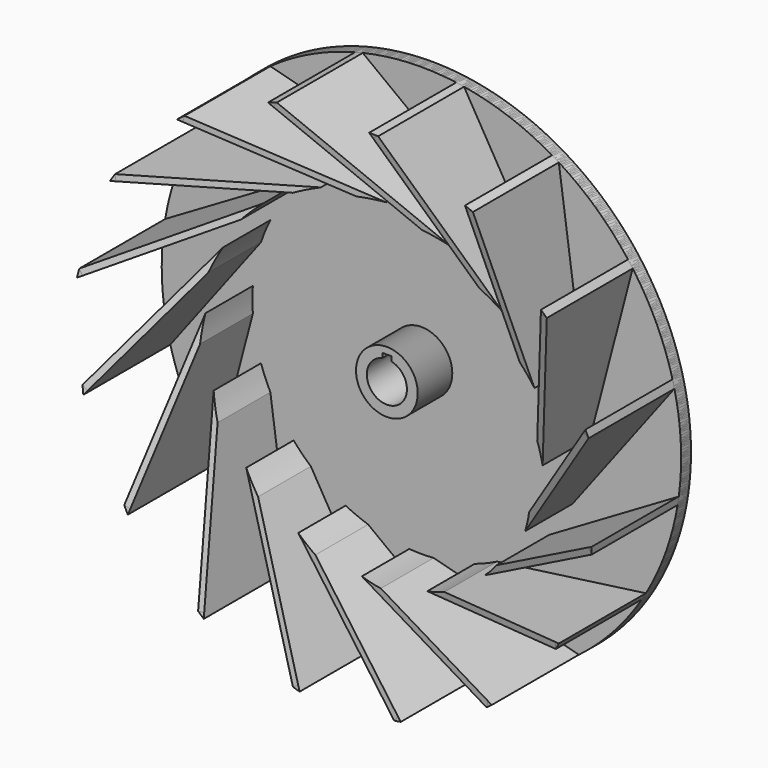
from build123d import *

# Parameters (mm, degrees)
F0_R      = 267.335
F0_R_2    = 20.6375
F1_DEPTH  = 12.7
F3_DEPTH  = 241.3
F2_R      = 31.75
F2_R_2    = 20.6375
F4_DEPTH  = 44.45
F7_DEPTH  = 6.35
F8_COUNT  = 16
F10_DEPTH = 57.15


# Not quite as in the source:
# - a feature names something its author has since deleted; it is built from what else it names


with BuildPart() as f1:
    # F0 (on Front) → F1 (new body)
    with BuildSketch(Plane.XZ):
        Circle(F0_R)
        Circle(F0_R_2, mode=Mode.SUBTRACT)
    extrude(amount=F1_DEPTH)

    # F2 (on face) → F3 (join)
    with BuildSketch(Plane.XZ.offset(12.7)):
        with BuildLine():
            Line((-162.0244501567, 212.6407293451), (-12.5453111688, 173.5371293634))
            ThreePointArc((-12.5453111688, 173.5371293634), (0, 173.99), (12.5453111688, 173.5371293634))
            Line((12.5453111688, 173.5371293634), (-155.4588853582, 217.4868667028))
            ThreePointArc((-155.4588853582, 217.4868667028), (-158.7601598142, 215.0888511308), (-162.0244501567, 212.6407293451))
        make_face()
    extrude(amount=F3_DEPTH)

    # F2 (on face) → F4 (join)
    with BuildSketch(Plane.XZ.offset(12.7)):
        Circle(F2_R)
        Circle(F2_R_2, mode=Mode.SUBTRACT)
    extrude(amount=F4_DEPTH)

    # F5 (on face) → F7 (cut, through all)
    with BuildSketch(Plane(origin=(43.2929607784, 0, 165.4935735946), x_dir=(0.9674446735, 0, -0.2530826025), z_dir=(0.2530826025, 0, 0.9674446735))):
        Polygon((-205.4400128284, -123.2503851183), (-205.4400128284, -254), (-31.7823338652, -254), (-31.7823338652, -73.66), align=None)
        Polygon((-210.5653604666, -124.714), (-210.5653604666, -254), (-205.4400128284, -254), (-205.4400128284, -123.2503851183), align=None)
    extrude(amount=-F7_DEPTH, mode=Mode.SUBTRACT)


with BuildPart() as f8_1:
    # F8: instance of F1
    add(f1.part.rotate(Axis((0, -75.4788592458, 0), (0, -1, 0)), 1 * 360 / F8_COUNT))


with BuildPart() as f8_2:
    # F8: instance of F1
    add(f1.part.rotate(Axis((0, -75.4788592458, 0), (0, -1, 0)), 2 * 360 / F8_COUNT))


with BuildPart() as f8_3:
    # F8: instance of F1
    add(f1.part.rotate(Axis((0, -75.4788592458, 0), (0, -1, 0)), 3 * 360 / F8_COUNT))


with BuildPart() as f8_4:
    # F8: instance of F1
    add(f1.part.rotate(Axis((0, -75.4788592458, 0), (0, -1, 0)), 4 * 360 / F8_COUNT))


with BuildPart() as f8_5:
    # F8: instance of F1
    add(f1.part.rotate(Axis((0, -75.4788592458, 0), (0, -1, 0)), 5 * 360 / F8_COUNT))


with BuildPart() as f8_6:
    # F8: instance of F1
    add(f1.part.rotate(Axis((0, -75.4788592458, 0), (0, -1, 0)), 6 * 360 / F8_COUNT))


with BuildPart() as f8_7:
    # F8: instance of F1
    add(f1.part.rotate(Axis((0, -75.4788592458, 0), (0, -1, 0)), 7 * 360 / F8_COUNT))


with BuildPart() as f8_8:
    # F8: instance of F1
    add(f1.part.rotate(Axis((0, -75.4788592458, 0), (0, -1, 0)), 8 * 360 / F8_COUNT))


with BuildPart() as f8_9:
    # F8: instance of F1
    add(f1.part.rotate(Axis((0, -75.4788592458, 0), (0, -1, 0)), 9 * 360 / F8_COUNT))


with BuildPart() as f8_10:
    # F8: instance of F1
    add(f1.part.rotate(Axis((0, -75.4788592458, 0), (0, -1, 0)), 10 * 360 / F8_COUNT))


with BuildPart() as f8_11:
    # F8: instance of F1
    add(f1.part.rotate(Axis((0, -75.4788592458, 0), (0, -1, 0)), 11 * 360 / F8_COUNT))


with BuildPart() as f8_12:
    # F8: instance of F1
    add(f1.part.rotate(Axis((0, -75.4788592458, 0), (0, -1, 0)), 12 * 360 / F8_COUNT))


with BuildPart() as f8_13:
    # F8: instance of F1
    add(f1.part.rotate(Axis((0, -75.4788592458, 0), (0, -1, 0)), 13 * 360 / F8_COUNT))


with BuildPart() as f8_14:
    # F8: instance of F1
    add(f1.part.rotate(Axis((0, -75.4788592458, 0), (0, -1, 0)), 14 * 360 / F8_COUNT))


with BuildPart() as f8_15:
    # F8: instance of F1
    add(f1.part.rotate(Axis((0, -75.4788592458, 0), (0, -1, 0)), 15 * 360 / F8_COUNT))


with BuildPart() as f10_tool:
    # F9 (on face) → F10 (new body, through all)
    with BuildSketch(Plane.XZ.offset(57.15)):
        with BuildLine():
            Line((-4.7625, 24.8539), (-4.7625, 20.0804631421))
            ThreePointArc((-4.7625, 20.0804631421), (0, 20.6375), (4.7625, 20.0804631421))
            Line((4.7625, 20.0804631421), (4.7625, 24.8539))
            Line((4.7625, 24.8539), (-4.7625, 24.8539))
        make_face()
    extrude(amount=-F10_DEPTH)


with BuildPart() as f1_1:
    add(f1.part)

    # F10: cut by f10_tool
    add(f10_tool.part, mode=Mode.SUBTRACT)


with BuildPart() as f8_1_1:
    add(f8_1.part)

    # F10: cut by f10_tool
    add(f10_tool.part, mode=Mode.SUBTRACT)


with BuildPart() as f8_2_1:
    add(f8_2.part)

    # F10: cut by f10_tool
    add(f10_tool.part, mode=Mode.SUBTRACT)


with BuildPart() as f8_3_1:
    add(f8_3.part)

    # F10: cut by f10_tool
    add(f10_tool.part, mode=Mode.SUBTRACT)


with BuildPart() as f8_4_1:
    add(f8_4.part)

    # F10: cut by f10_tool
    add(f10_tool.part, mode=Mode.SUBTRACT)


with BuildPart() as f8_5_1:
    add(f8_5.part)

    # F10: cut by f10_tool
    add(f10_tool.part, mode=Mode.SUBTRACT)


with BuildPart() as f8_6_1:
    add(f8_6.part)

    # F10: cut by f10_tool
    add(f10_tool.part, mode=Mode.SUBTRACT)


with BuildPart() as f8_7_1:
    add(f8_7.part)

    # F10: cut by f10_tool
    add(f10_tool.part, mode=Mode.SUBTRACT)


with BuildPart() as f8_8_1:
    add(f8_8.part)

    # F10: cut by f10_tool
    add(f10_tool.part, mode=Mode.SUBTRACT)


with BuildPart() as f8_9_1:
    add(f8_9.part)

    # F10: cut by f10_tool
    add(f10_tool.part, mode=Mode.SUBTRACT)


with BuildPart() as f8_10_1:
    add(f8_10.part)

    # F10: cut by f10_tool
    add(f10_tool.part, mode=Mode.SUBTRACT)


with BuildPart() as f8_11_1:
    add(f8_11.part)

    # F10: cut by f10_tool
    add(f10_tool.part, mode=Mode.SUBTRACT)


with BuildPart() as f8_12_1:
    add(f8_12.part)

    # F10: cut by f10_tool
    add(f10_tool.part, mode=Mode.SUBTRACT)


with BuildPart() as f8_13_1:
    add(f8_13.part)

    # F10: cut by f10_tool
    add(f10_tool.part, mode=Mode.SUBTRACT)


with BuildPart() as f8_14_1:
    add(f8_14.part)

    # F10: cut by f10_tool
    add(f10_tool.part, mode=Mode.SUBTRACT)


with BuildPart() as f8_15_1:
    add(f8_15.part)

    # F10: cut by f10_tool
    add(f10_tool.part, mode=Mode.SUBTRACT)


solid = Compound([f1_1.part, f8_1_1.part, f8_2_1.part, f8_3_1.part, f8_4_1.part, f8_5_1.part, f8_6_1.part, f8_7_1.part, f8_8_1.part, f8_9_1.part, f8_10_1.part, f8_11_1.part, f8_12_1.part, f8_13_1.part, f8_14_1.part, f8_15_1.part])
